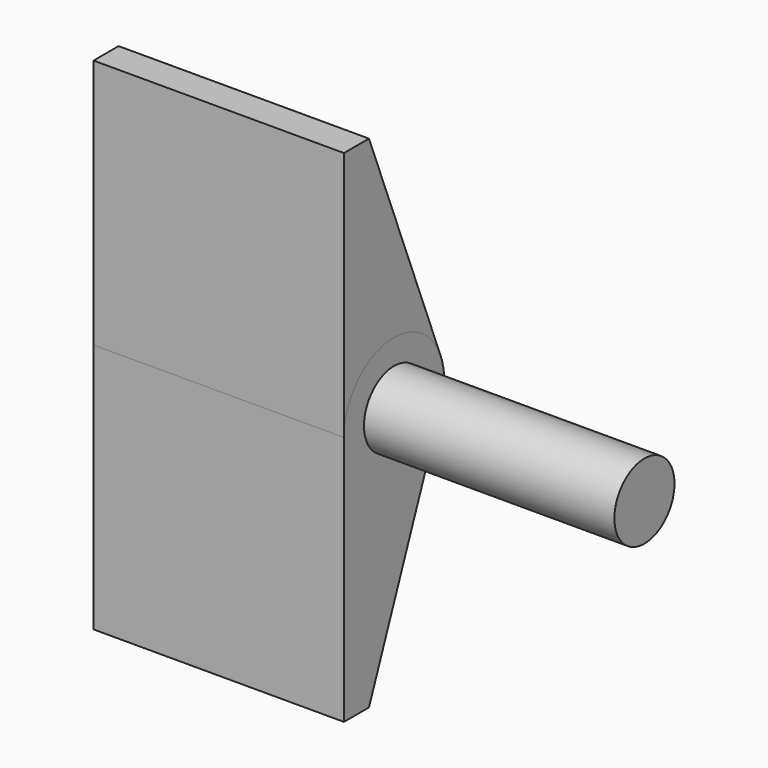
from build123d import *

# Parameters (mm, degrees)
F1_DEPTH = 40
F2_R     = 6
F3_DEPTH = 40.001
F5_DEPTH = 40
F6_R     = 6
F7_DEPTH = 40


with BuildPart() as f1:
    # F0 (on Right) → F1 (new body)
    with BuildSketch(Plane.YZ):
        with BuildLine():
            ThreePointArc((-10, 0), (0, -10), (10, 0))
            ThreePointArc((10, 0), (9.8246940609, 1.8642388822), (9.304922678, 3.6631153348))
            ThreePointArc((9.304922678, 3.6631153348), (-1.8642388822, 9.8246940609), (-10, 0))
        make_face()
        with BuildLine():
            ThreePointArc((-10, 0), (-1.8642388822, 9.8246940609), (9.304922678, 3.6631153348))
            Line((9.304922678, 3.6631153348), (-5, 40))
            Line((-5, 40), (-10, 40))
            Line((-10, 40), (-10, 0))
        make_face()
    extrude(amount=F1_DEPTH)

    # F2 (on face) → F3 (cut, through all)
    with BuildSketch(Plane.YZ.offset(40)):
        Circle(F2_R)
    extrude(amount=-F3_DEPTH, mode=Mode.SUBTRACT)


with BuildPart() as f5:
    # F4 (on Right) → F5 (new body)
    with BuildSketch(Plane.YZ):
        with BuildLine():
            ThreePointArc((9.304922678, -3.6631153348), (9.8246940609, -1.8642388822), (10, 0))
            ThreePointArc((10, 0), (0, 10), (-10, 0))
            ThreePointArc((-10, 0), (-1.8642388822, -9.8246940609), (9.304922678, -3.6631153348))
        make_face()
        with BuildLine():
            ThreePointArc((9.304922678, -3.6631153348), (-1.8642388822, -9.8246940609), (-10, 0))
            Line((-10, 0), (-10, -40))
            Line((-10, -40), (-5, -40))
            Line((-5, -40), (9.304922678, -3.6631153348))
        make_face()
    extrude(amount=F5_DEPTH)

    # F6 (on face) → F7 (join)
    with BuildSketch(Plane.YZ.offset(40)):
        Circle(F6_R)
    extrude(amount=F7_DEPTH)


solid = Compound([f1.part, f5.part])
